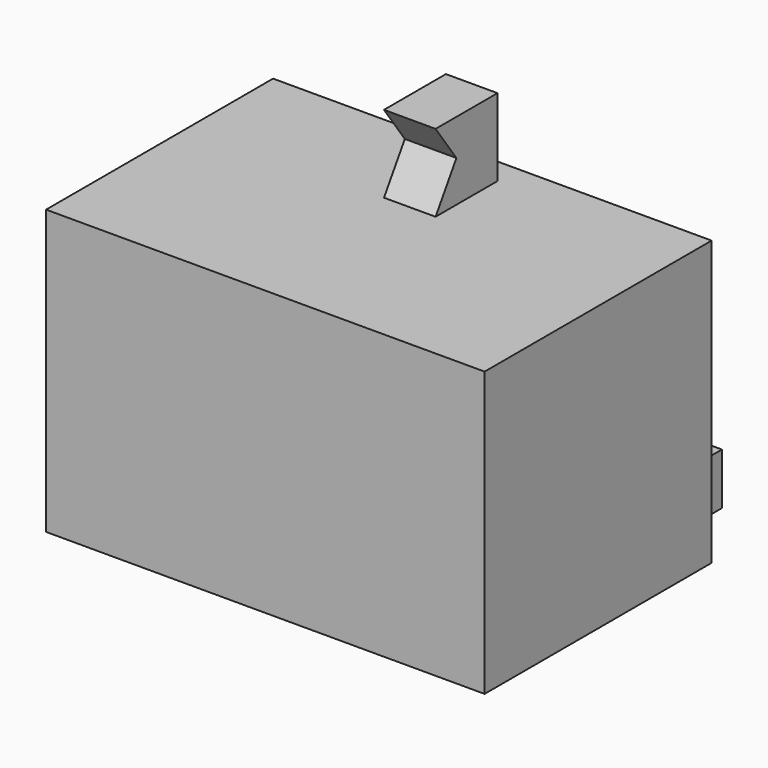
from build123d import *

# Parameters (mm, degrees)
F0_W      = 17
F0_H      = 11
F1_DEPTH  = 11
F3_DEPTH  = 10
F4_W      = 13
F4_H      = 2
F5_DEPTH  = 3
F6_W      = 1.5
F6_H      = 1.5
F7_DEPTH  = 15.001
F8_W      = 2
F8_H      = 2
F9_DEPTH  = 3
F11_DEPTH = 9.501
F12_DEPTH = 1


# Not quite as in the source:
# - a feature names something its author has since deleted; it is built from what else it names


with BuildPart() as f1:
    # F0 (on Top) → F1 (new body)
    with BuildSketch(Plane.XY):
        with Locations((1.3527604751, 0)):
            Rectangle(F0_W, F0_H)
    extrude(amount=F1_DEPTH)

    # F2 (on face) → F3 (cut)
    with BuildSketch(Plane(origin=(0, 5.5, 0), x_dir=(-1, 0, 0), z_dir=(0, 1, 0))):
        Polygon((-7.8527604751, 2), (-1.3527604751, 2), (5.1472395249, 2), (5.1472395249, 5.5), (5.1472395249, 9), (-1.3527604751, 9), (-7.8527604751, 9), (-7.8527604751, 5.5), align=None)
    extrude(amount=-F3_DEPTH, mode=Mode.SUBTRACT)

    # F4 (on face) → F5 (join)
    with BuildSketch(Plane(origin=(0, 5.5, 0), x_dir=(-1, 0, 0), z_dir=(0, 1, 0))):
        with Locations((-1.3527604751, 1)):
            Rectangle(F4_W, F4_H)
    extrude(amount=F5_DEPTH)

    # F6 (on face) → F7 (cut, through all)
    with BuildSketch(Plane.YZ.offset(7.8527604751)):
        with Locations((7, 1)):
            Rectangle(F6_W, F6_H)
    extrude(amount=-F7_DEPTH, mode=Mode.SUBTRACT)

    # F8 (on face) → F9 (join)
    with BuildSketch(Plane.XY.offset(11)):
        with Locations((1.3527604751, 2.5)):
            Rectangle(F8_W, F8_H)
    extrude(amount=F9_DEPTH)

    # F10 (on face) → F11 (cut, through all)
    with BuildSketch(Plane.YZ.offset(2.3527604751)):
        Polygon((2.5089287665, 12.594983913), (1.5, 14), (1.5, 11), align=None)
    extrude(amount=-F11_DEPTH, mode=Mode.SUBTRACT)

    # F12 (add): a face of the model
    f12_faces = [f1.faces().sort_by_distance(p)[0] for p in [
        (1.3527604751, 3.5, 12.5),
    ]]
    extrude(f12_faces, amount=F12_DEPTH)


solid = f1.part
